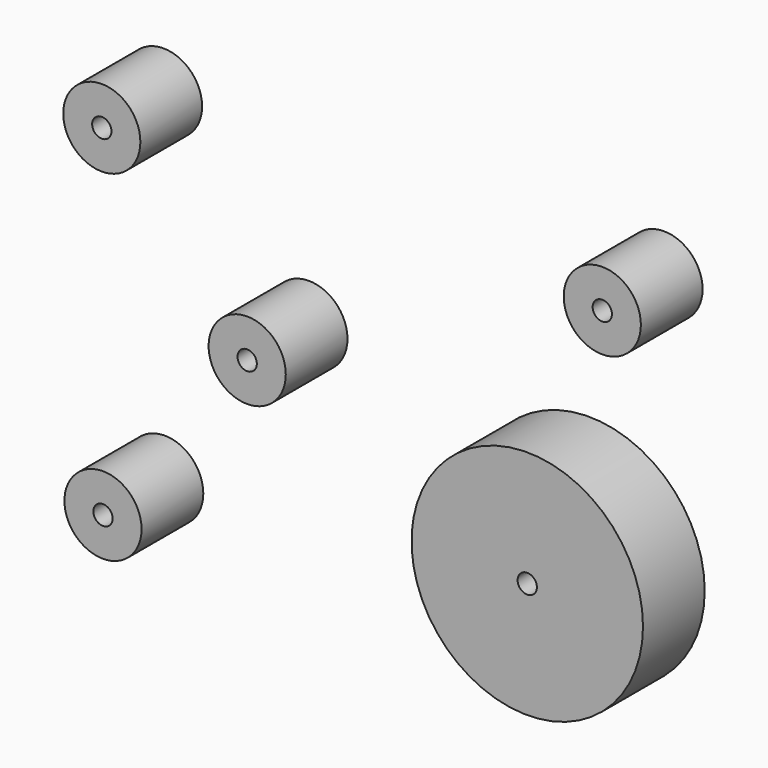
from build123d import *

# Parameters (mm, degrees)
F0_R       = 25.4
F2_DEPTH   = 50.8
F1_R       = 76.2
F5_DEPTH   = 50.8
F6_D       = 12.7
F6_2_D     = 12.7
F6_3_D     = 12.7
F6_ON_F1_D = 12.7
F7_D       = 12.7


# Not quite as in the source:
# - the program builds the solid bodies; features that only make, move or delete a surface that nothing else refers to are left out


with BuildPart() as f2:
    # F0 (on Front) → F2 (new body)
    with BuildSketch(Plane.XZ):
        with Locations((-316.3281083107, 152.4865627289)):
            Circle(F0_R)
    extrude(amount=F2_DEPTH)

    # F6 (through all)
    with Locations(Plane(origin=(0, 0, 0), x_dir=(1, 0, 0), z_dir=(0, 1, 0))):
        with Locations((-315.5324161053, 71.7213749886), (-316.3281083107, -152.4865627289), (13.2203800604, -153.6489874125), (-220.5883562565, -48.8537736237)):
            Hole(F6_D / 2)


with BuildPart() as f2b:
    # F0 (on Front) → F2, piece 2 (new body)
    with BuildSketch(Plane.XZ):
        with Locations((-315.5324161053, -71.7213749886)):
            Circle(F0_R)
    extrude(amount=F2_DEPTH)

    # F6#2 (through all)
    with Locations(Plane(origin=(0, 0, 0), x_dir=(1, 0, 0), z_dir=(0, 1, 0))):
        with Locations((-315.5324161053, 71.7213749886), (-316.3281083107, -152.4865627289), (13.2203800604, -153.6489874125), (-220.5883562565, -48.8537736237)):
            Hole(F6_2_D / 2)


with BuildPart() as f2c:
    # F0 (on Front) → F2, piece 3 (new body)
    with BuildSketch(Plane.XZ):
        with Locations((13.2203800604, 153.6489874125)):
            Circle(F0_R)
    extrude(amount=F2_DEPTH)

    # F6#3 (through all)
    with Locations(Plane(origin=(0, 0, 0), x_dir=(1, 0, 0), z_dir=(0, 1, 0))):
        with Locations((-315.5324161053, 71.7213749886), (-316.3281083107, -152.4865627289), (13.2203800604, -153.6489874125), (-220.5883562565, -48.8537736237)):
            Hole(F6_3_D / 2)


with BuildPart() as f2d:
    # F1 (on Front) → F2, piece 4 (new body)
    with BuildSketch(Plane.XZ):
        with Locations((-36.1828282475, -20.7152944058)):
            Circle(F1_R)
    extrude(amount=F2_DEPTH)

    # F6 on F1 (through all)
    with Locations(Plane(origin=(0, 0, 0), x_dir=(1, 0, 0), z_dir=(0, 1, 0))):
        with Locations((-36.1828282475, 20.7152944058)):
            Hole(F6_ON_F1_D / 2)


with BuildPart() as f5:
    # F0 (on Front) → F5 (new body)
    with BuildSketch(Plane.XZ):
        with Locations((-220.5883562565, 48.8537736237)):
            Circle(F0_R)
    extrude(amount=F5_DEPTH)

    # F7 (through all)
    with Locations(Plane(origin=(0, 0, 0), x_dir=(1, 0, 0), z_dir=(0, 1, 0))):
        with Locations((-220.5883562565, -48.8537736237)):
            Hole(F7_D / 2)


solid = Compound([f2.part, f2b.part, f2c.part, f2d.part, f5.part])
